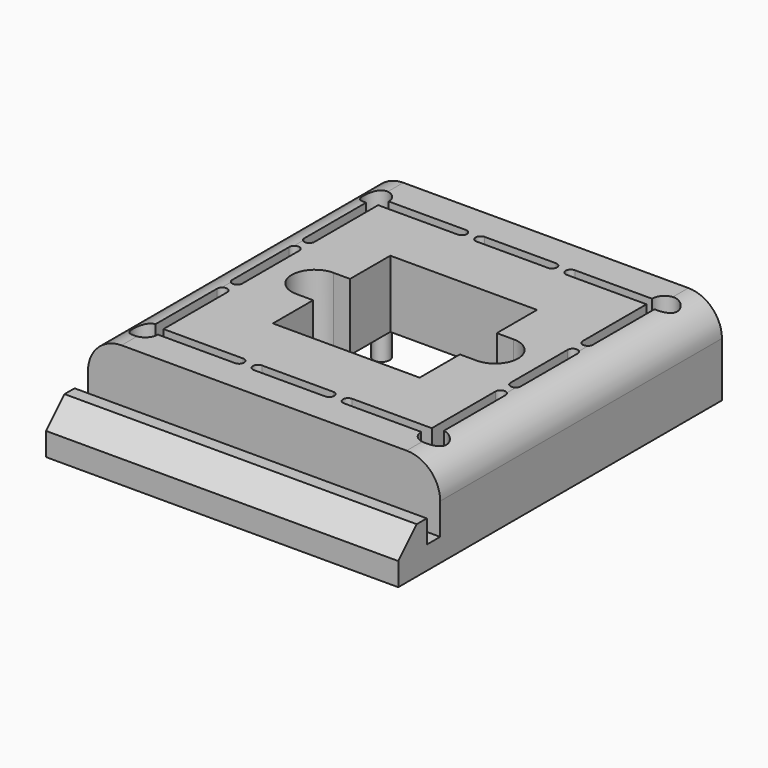
from build123d import *

# Parameters (mm, degrees)
F0_W        = 39
F0_H        = 39
F0_R        = 0.975
F1_DEPTH    = 9
F2_T1_DEPTH = 62
F4_DEPTH    = 21
F5_DEPTH    = 21
F6_DEPTH    = 5.5
F7_DEPTH    = 1.5
F8_DEPTH    = 2.5
F9_DEPTH    = 1.5
F10_R       = 1.25
F11_DEPTH   = 2.5
F12_DEPTH   = 5
F13_DEPTH   = 1


# Not quite as in the source:
# - a fillet or chamfer that OpenCascade refuses, or shapes differently, is made with other operations: its cross-section is extruded or revolved along the edge and cut away or added


with BuildPart() as f1:
    # F0 (on Top) → F1 (new body)
    with BuildSketch(Plane.XY):
        Polygon((-2.625, 21), (-21, 21), (-21, -21), (-2.625, -21), (2.625, -21), (21, -21), (21, 21), (2.625, 21), align=None)
        Rectangle(F0_W, F0_H, mode=Mode.SUBTRACT)
        Rectangle(F0_W, F0_H)
        with BuildLine():
            ThreePointArc((16, 4.25), (16.6, 4.85), (17.2, 4.25))
            Line((17.2, 4.25), (17.2, -4.25))
            ThreePointArc((17.2, -4.25), (16.6, -4.85), (16, -4.25))
            Line((16, -4.25), (16, -6.5))
            ThreePointArc((16, -6.5), (16.6, -5.9), (17.2, -6.5))
            Line((17.2, -6.5), (17.2, -15.7))
            ThreePointArc((17.2, -15.7), (18.2606601718, -18.2606601718), (15.7, -17.2))
            Line((15.7, -17.2), (6.5, -17.2))
            ThreePointArc((6.5, -17.2), (5.9, -16.6), (6.5, -16))
            Line((6.5, -16), (4.25, -16))
            ThreePointArc((4.25, -16), (4.85, -16.6), (4.25, -17.2))
            Line((4.25, -17.2), (-4.25, -17.2))
            ThreePointArc((-4.25, -17.2), (-4.85, -16.6), (-4.25, -16))
            Line((-4.25, -16), (-6.5, -16))
            ThreePointArc((-6.5, -16), (-5.9, -16.6), (-6.5, -17.2))
            Line((-6.5, -17.2), (-15.7, -17.2))
            ThreePointArc((-15.7, -17.2), (-18.2606601718, -18.2606601718), (-17.2, -15.7))
            Line((-17.2, -15.7), (-17.2, -6.5))
            ThreePointArc((-17.2, -6.5), (-16.6, -5.9), (-16, -6.5))
            Line((-16, -6.5), (-16, -4.25))
            ThreePointArc((-16, -4.25), (-16.6, -4.85), (-17.2, -4.25))
            Line((-17.2, -4.25), (-17.2, 4.25))
            ThreePointArc((-17.2, 4.25), (-16.6, 4.85), (-16, 4.25))
            Line((-16, 4.25), (-16, 6.5))
            ThreePointArc((-16, 6.5), (-16.6, 5.9), (-17.2, 6.5))
            Line((-17.2, 6.5), (-17.2, 15.7))
            ThreePointArc((-17.2, 15.7), (-18.2606601718, 18.2606601718), (-15.7, 17.2))
            Line((-15.7, 17.2), (-6.5, 17.2))
            ThreePointArc((-6.5, 17.2), (-5.9, 16.6), (-6.5, 16))
            Line((-6.5, 16), (-4.25, 16))
            ThreePointArc((-4.25, 16), (-4.85, 16.6), (-4.25, 17.2))
            Line((-4.25, 17.2), (4.25, 17.2))
            ThreePointArc((4.25, 17.2), (4.85, 16.6), (4.25, 16))
            Line((4.25, 16), (6.5, 16))
            ThreePointArc((6.5, 16), (5.9, 16.6), (6.5, 17.2))
            Line((6.5, 17.2), (15.7, 17.2))
            ThreePointArc((15.7, 17.2), (18.2606601718, 18.2606601718), (17.2, 15.7))
            Line((17.2, 15.7), (17.2, 6.5))
            ThreePointArc((17.2, 6.5), (16.6, 5.9), (16, 6.5))
            Line((16, 6.5), (16, 4.25))
        make_face(mode=Mode.SUBTRACT)
        Polygon((16, -4.25), (16, 4.25), (16, 6.5), (16, 16), (6.5, 16), (4.25, 16), (-4.25, 16), (-6.5, 16), (-16, 16), (-16, 6.5), (-16, 4.25), (-16, -4.25), (-16, -6.5), (-16, -16), (-6.5, -16), (-4.25, -16), (4.25, -16), (6.5, -16), (16, -16), (16, -6.5), align=None)
        with Locations((-14, -14)):
            Circle(F0_R, mode=Mode.SUBTRACT)
        with Locations((14, -14)):
            Circle(F0_R, mode=Mode.SUBTRACT)
        with Locations((-14, 14)):
            Circle(F0_R, mode=Mode.SUBTRACT)
        Polygon((-8.75, 14), (0, 14), (0, 10.75), (-8.75, 10.75), (-9.75, 10.75), (-9.75, 14), align=None, mode=Mode.SUBTRACT)
        with BuildLine():
            Line((-8.75, 8.75), (8.75, 8.75))
            Line((8.75, 8.75), (8.75, 2.75))
            Line((8.75, 2.75), (10.75, 2.75))
            ThreePointArc((10.75, 2.75), (13.5, 0), (10.75, -2.75))
            Line((10.75, -2.75), (8.75, -2.75))
            Line((8.75, -2.75), (8.75, -8.75))
            Line((8.75, -8.75), (-8.75, -8.75))
            Line((-8.75, -8.75), (-8.75, -2.75))
            Line((-8.75, -2.75), (-10.75, -2.75))
            ThreePointArc((-10.75, -2.75), (-13.5, 0), (-10.75, 2.75))
            Line((-10.75, 2.75), (-8.75, 2.75))
            Line((-8.75, 2.75), (-8.75, 8.75))
        make_face(mode=Mode.SUBTRACT)
        Polygon((10.75, 3.8126846775), (10.75, 8.75), (10.75, 9.75), (14, 9.75), (14, 8.75), (14, 3.8126846775), align=None, mode=Mode.SUBTRACT)
        with Locations((14, 14)):
            Circle(F0_R, mode=Mode.SUBTRACT)
        Polygon((0, 10.75), (0, 14), (-8.75, 14), (-9.75, 14), (-9.75, 10.75), (-8.75, 10.75), align=None)
        Polygon((10.75, 9.75), (10.75, 8.75), (10.75, 3.8126846775), (14, 3.8126846775), (14, 8.75), (14, 9.75), align=None)
        with Locations((14, -14)):
            Circle(F0_R)
        with Locations((-14, -14)):
            Circle(F0_R)
        with Locations((-14, 14)):
            Circle(F0_R)
        with Locations((14, 14)):
            Circle(F0_R)
    extrude(amount=F1_DEPTH)

    # F2: fillet of radius 4 on 2 edges, made by hand

    # F2_s2 → F2_t1 (cut)
    with BuildSketch(Plane.XZ.offset(-31)):
        with BuildLine():
            ThreePointArc((-21, 5), (-19.8284271247, 7.8284271247), (-17, 9))
            Line((-17, 9), (-21, 9))
            Line((-21, 9), (-21, 5))
        make_face()
        with BuildLine():
            ThreePointArc((21, 5), (19.8284271247, 7.8284271247), (17, 9))
            Line((17, 9), (21, 9))
            Line((21, 9), (21, 5))
        make_face()
    extrude(amount=F2_T1_DEPTH, mode=Mode.SUBTRACT)

    # F3 (on Right) → F4 (join)
    with BuildSketch(Plane.YZ):
        Polygon((-21, 0), (-21, 1.25), (-23, 1.25), (-23, 4), (-24.5, 4), (-27.25, 1.25), (-27.25, -1.5), (-23, -1.5), (-21, -1.5), align=None)
    extrude(amount=F4_DEPTH)

    # F5 (add): a face of the model
    f5_faces = [f1.faces().sort_by_distance(p)[0] for p in [
        (0, -24.2579908676, 0.6723744292),
    ]]
    extrude(f5_faces, amount=F5_DEPTH)

    # F0 (on Top) → F6 (join)
    with BuildSketch(Plane.XY):
        with Locations((-14, -14)):
            Circle(F0_R)
        with Locations((14, -14)):
            Circle(F0_R)
        with Locations((-14, 14)):
            Circle(F0_R)
        with Locations((14, 14)):
            Circle(F0_R)
    extrude(amount=-F6_DEPTH)

    # F0 (on Top) → F7 (join)
    with BuildSketch(Plane.XY):
        Rectangle(F0_W, F0_H)
        with BuildLine():
            ThreePointArc((16, 4.25), (16.6, 4.85), (17.2, 4.25))
            Line((17.2, 4.25), (17.2, -4.25))
            ThreePointArc((17.2, -4.25), (16.6, -4.85), (16, -4.25))
            Line((16, -4.25), (16, -6.5))
            ThreePointArc((16, -6.5), (16.6, -5.9), (17.2, -6.5))
            Line((17.2, -6.5), (17.2, -15.7))
            ThreePointArc((17.2, -15.7), (18.2606601718, -18.2606601718), (15.7, -17.2))
            Line((15.7, -17.2), (6.5, -17.2))
            ThreePointArc((6.5, -17.2), (5.9, -16.6), (6.5, -16))
            Line((6.5, -16), (4.25, -16))
            ThreePointArc((4.25, -16), (4.85, -16.6), (4.25, -17.2))
            Line((4.25, -17.2), (-4.25, -17.2))
            ThreePointArc((-4.25, -17.2), (-4.85, -16.6), (-4.25, -16))
            Line((-4.25, -16), (-6.5, -16))
            ThreePointArc((-6.5, -16), (-5.9, -16.6), (-6.5, -17.2))
            Line((-6.5, -17.2), (-15.7, -17.2))
            ThreePointArc((-15.7, -17.2), (-18.2606601718, -18.2606601718), (-17.2, -15.7))
            Line((-17.2, -15.7), (-17.2, -6.5))
            ThreePointArc((-17.2, -6.5), (-16.6, -5.9), (-16, -6.5))
            Line((-16, -6.5), (-16, -4.25))
            ThreePointArc((-16, -4.25), (-16.6, -4.85), (-17.2, -4.25))
            Line((-17.2, -4.25), (-17.2, 4.25))
            ThreePointArc((-17.2, 4.25), (-16.6, 4.85), (-16, 4.25))
            Line((-16, 4.25), (-16, 6.5))
            ThreePointArc((-16, 6.5), (-16.6, 5.9), (-17.2, 6.5))
            Line((-17.2, 6.5), (-17.2, 15.7))
            ThreePointArc((-17.2, 15.7), (-18.2606601718, 18.2606601718), (-15.7, 17.2))
            Line((-15.7, 17.2), (-6.5, 17.2))
            ThreePointArc((-6.5, 17.2), (-5.9, 16.6), (-6.5, 16))
            Line((-6.5, 16), (-4.25, 16))
            ThreePointArc((-4.25, 16), (-4.85, 16.6), (-4.25, 17.2))
            Line((-4.25, 17.2), (4.25, 17.2))
            ThreePointArc((4.25, 17.2), (4.85, 16.6), (4.25, 16))
            Line((4.25, 16), (6.5, 16))
            ThreePointArc((6.5, 16), (5.9, 16.6), (6.5, 17.2))
            Line((6.5, 17.2), (15.7, 17.2))
            ThreePointArc((15.7, 17.2), (18.2606601718, 18.2606601718), (17.2, 15.7))
            Line((17.2, 15.7), (17.2, 6.5))
            ThreePointArc((17.2, 6.5), (16.6, 5.9), (16, 6.5))
            Line((16, 6.5), (16, 4.25))
        make_face(mode=Mode.SUBTRACT)
    extrude(amount=-F7_DEPTH)

    # F8 (cut): a face of the model
    f8_faces = [f1.faces().sort_by_distance(p)[0] for p in [
        (-18.9484567107, 0, -1.5),
    ]]
    extrude(f8_faces, amount=-F8_DEPTH, mode=Mode.SUBTRACT)

    # F0 (on Top) → F9 (join)
    with BuildSketch(Plane.XY):
        Polygon((-2.625, 21), (-21, 21), (-21, -21), (-2.625, -21), (2.625, -21), (21, -21), (21, 21), (2.625, 21), align=None)
        Rectangle(F0_W, F0_H, mode=Mode.SUBTRACT)
    extrude(amount=-F9_DEPTH)

    # F10 (on face) → F11 (cut)
    with BuildSketch(Plane(origin=(0, 0, -1.5), x_dir=(1, 0, 0), z_dir=(0, 0, -1))):
        with Locations((10.5, 24.75)):
            Circle(F10_R)
        with Locations((0, 24.75)):
            Circle(F10_R)
        with Locations((-10.5, 24.75)):
            Circle(F10_R)
    extrude(amount=-F11_DEPTH, mode=Mode.SUBTRACT)

    # F0 (on Top) → F12 (cut)
    with BuildSketch(Plane.XY):
        Polygon((10.75, 9.75), (10.75, 8.75), (10.75, 3.8126846775), (14, 3.8126846775), (14, 8.75), (14, 9.75), align=None)
        Polygon((0, 10.75), (0, 14), (-8.75, 14), (-9.75, 14), (-9.75, 10.75), (-8.75, 10.75), align=None)
    extrude(amount=F12_DEPTH, mode=Mode.SUBTRACT)

    # F0 (on Top) → F13 (cut)
    with BuildSketch(Plane.XY):
        Polygon((16, -4.25), (16, 4.25), (16, 6.5), (16, 16), (6.5, 16), (4.25, 16), (-4.25, 16), (-6.5, 16), (-16, 16), (-16, 6.5), (-16, 4.25), (-16, -4.25), (-16, -6.5), (-16, -16), (-6.5, -16), (-4.25, -16), (4.25, -16), (6.5, -16), (16, -16), (16, -6.5), align=None)
        with Locations((-14, -14)):
            Circle(F0_R, mode=Mode.SUBTRACT)
        with Locations((14, -14)):
            Circle(F0_R, mode=Mode.SUBTRACT)
        with Locations((-14, 14)):
            Circle(F0_R, mode=Mode.SUBTRACT)
        Polygon((-8.75, 14), (0, 14), (0, 10.75), (-8.75, 10.75), (-9.75, 10.75), (-9.75, 14), align=None, mode=Mode.SUBTRACT)
        with BuildLine():
            Line((-8.75, 8.75), (8.75, 8.75))
            Line((8.75, 8.75), (8.75, 2.75))
            Line((8.75, 2.75), (10.75, 2.75))
            ThreePointArc((10.75, 2.75), (13.5, 0), (10.75, -2.75))
            Line((10.75, -2.75), (8.75, -2.75))
            Line((8.75, -2.75), (8.75, -8.75))
            Line((8.75, -8.75), (-8.75, -8.75))
            Line((-8.75, -8.75), (-8.75, -2.75))
            Line((-8.75, -2.75), (-10.75, -2.75))
            ThreePointArc((-10.75, -2.75), (-13.5, 0), (-10.75, 2.75))
            Line((-10.75, 2.75), (-8.75, 2.75))
            Line((-8.75, 2.75), (-8.75, 8.75))
        make_face(mode=Mode.SUBTRACT)
        Polygon((10.75, 3.8126846775), (10.75, 8.75), (10.75, 9.75), (14, 9.75), (14, 8.75), (14, 3.8126846775), align=None, mode=Mode.SUBTRACT)
        with Locations((14, 14)):
            Circle(F0_R, mode=Mode.SUBTRACT)
    extrude(amount=F13_DEPTH, mode=Mode.SUBTRACT)


solid = f1.part
